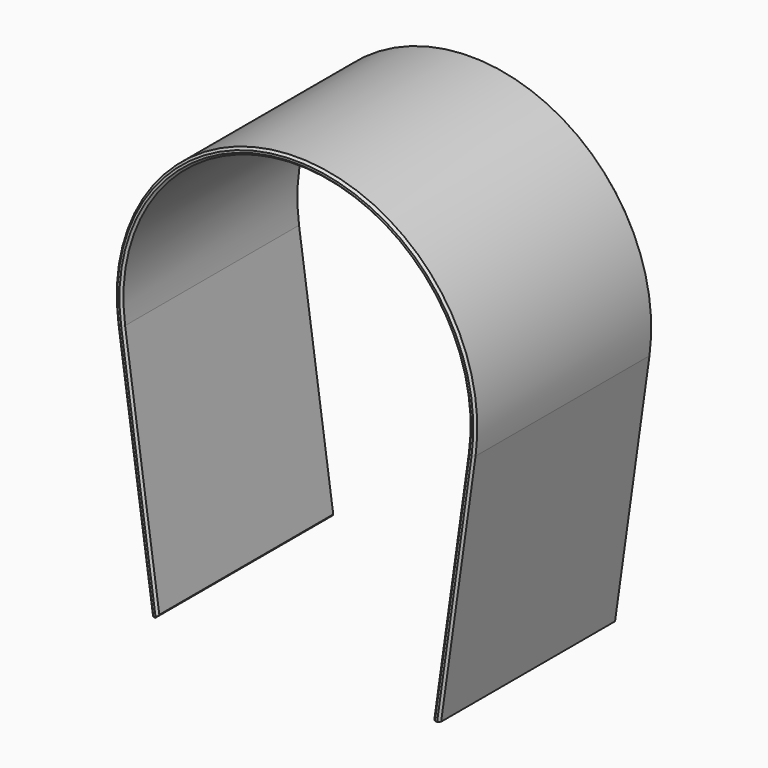
from build123d import *

# Parameters (mm, degrees)
F1_DEPTH     = 100
F2_T1_DEPTH  = 105.8849898869
F2_T3_DEPTH  = 114.5074829388
F2_T5_DEPTH  = 114.0858604347
F2_T7_DEPTH  = 114.5074829388
F2_T9_DEPTH  = 114.0858604347
F2_T12_ANGLE = 196
F2_T14_ANGLE = 196
F2_T16_ANGLE = 196
F2_T18_ANGLE = 196


# Not quite as in the source:
# - a fillet or chamfer that OpenCascade refuses, or shapes differently, is made with other operations: its cross-section is extruded or revolved along the edge and cut away or added


with BuildPart() as f1:
    # F0 (on Front) → F1 (new body)
    with BuildSketch(Plane.XZ):
        with BuildLine():
            Line((-61.9215476124, -110.8464484404), (-77.5, 0))
            ThreePointArc((-77.5, 0), (0, 89.1535515596), (77.5, 0))
            Line((77.5, 0), (61.9215476124, -110.8464484404))
            Line((61.9215476124, -110.8464484404), (64.95103033, -110.8464484404))
            Line((64.95103033, -110.8464484404), (80.4708042062, -0.4175193029))
            ThreePointArc((80.4708042062, -0.4175193029), (0, 92.1535515596), (-80.4708042062, -0.4175193029))
            Line((-80.4708042062, -0.4175193029), (-64.95103033, -110.8464484404))
            Line((-64.95103033, -110.8464484404), (-61.9215476124, -110.8464484404))
        make_face()
    extrude(amount=F1_DEPTH)

    # F2: chamfer of 1 on 17 edges, made by hand

    # F2_s2 → F2_t1 (cut)
    with BuildSketch(Plane.XZ.offset(-2.9424949434)):
        Polygon((-63.0719160196, -110.8464484404), (-62.0816479509, -109.7072753394), (-61.9215476124, -110.8464484404), align=None)
    extrude(amount=F2_T1_DEPTH, mode=Mode.SUBTRACT)

    # F2_s4 → F2_t3 (cut)
    with BuildSketch(Plane(origin=(14.4352522013, 0, -102.7121564484), x_dir=(0, 1, 0), z_dir=(-0.139173101, 0, 0.9902680687))):
        Polygon((-1, 76.7457753275), (0, 77.7457753275), (0, 76.7457753275), align=None)
        Polygon((-99, 76.7457753275), (-100, 77.7457753275), (-100, 76.7457753275), align=None)
    extrude(amount=F2_T3_DEPTH, mode=Mode.SUBTRACT)

    # F2_s6 → F2_t5 (cut)
    with BuildSketch(Plane(origin=(-1.5011092824, 0, 10.6809475379), x_dir=(0, 1, 0), z_dir=(0.139173101, 0, -0.9902680687))):
        Polygon((-1, -79.7457753275), (0, -78.7457753275), (0, -79.7457753275), align=None)
        Polygon((-99, -79.7457753275), (-100, -78.7457753275), (-100, -79.7457753275), align=None)
    extrude(amount=F2_T5_DEPTH, mode=Mode.SUBTRACT)

    # F2_s8 → F2_t7 (cut)
    with BuildSketch(Plane(origin=(1.5011092824, 0, 10.6809475379), x_dir=(0, 1, 0), z_dir=(-0.139173101, 0, -0.9902680687))):
        Polygon((-1, 76.7457753275), (0, 77.7457753275), (0, 76.7457753275), align=None)
        Polygon((-99, 76.7457753275), (-100, 77.7457753275), (-100, 76.7457753275), align=None)
    extrude(amount=F2_T7_DEPTH, mode=Mode.SUBTRACT)

    # F2_s10 → F2_t9 (cut)
    with BuildSketch(Plane(origin=(-14.37657369, 0, -102.2946371455), x_dir=(0, 1, 0), z_dir=(0.139173101, 0, 0.9902680687))):
        Polygon((-1, -79.7457753275), (0, -78.7457753275), (0, -79.7457753275), align=None)
        Polygon((-99, -79.7457753275), (-100, -78.7457753275), (-100, -79.7457753275), align=None)
    extrude(amount=F2_T9_DEPTH, mode=Mode.SUBTRACT)

    # F2_s11 → F2_t12 (revolve, cut)
    with BuildSketch(Plane(origin=(1.5011092824, 0, 10.6809475379), x_dir=(0, 1, 0), z_dir=(-0.139173101, 0, -0.9902680687))):
        Polygon((-1, 79.7457753275), (0, 78.7457753275), (0, 79.7457753275), align=None)
    revolve(axis=Axis((0, 0, 10.8919146894), (0, -1, 0)), revolution_arc=F2_T12_ANGLE, mode=Mode.SUBTRACT)

    # F2_s13 → F2_t14 (revolve, cut)
    with BuildSketch(Plane(origin=(1.5011092824, 0, 10.6809475379), x_dir=(0, 1, 0), z_dir=(-0.139173101, 0, -0.9902680687))):
        Polygon((-99, 79.7457753275), (-100, 78.7457753275), (-100, 79.7457753275), align=None)
    revolve(axis=Axis((0, -100, 10.8919146894), (0, -1, 0)), revolution_arc=F2_T14_ANGLE, mode=Mode.SUBTRACT)

    # F2_s15 → F2_t16 (revolve, cut)
    with BuildSketch(Plane(origin=(-1.5011092824, 0, 10.6809475379), x_dir=(0, 1, 0), z_dir=(0.139173101, 0, -0.9902680687))):
        Polygon((-1, -76.7457753275), (0, -77.7457753275), (0, -76.7457753275), align=None)
    revolve(axis=Axis((0, 0, 10.8919146894), (0, 1, 0)), revolution_arc=F2_T16_ANGLE, mode=Mode.SUBTRACT)

    # F2_s17 → F2_t18 (revolve, cut)
    with BuildSketch(Plane(origin=(-1.5011092824, 0, 10.6809475379), x_dir=(0, 1, 0), z_dir=(0.139173101, 0, -0.9902680687))):
        Polygon((-99, -76.7457753275), (-100, -77.7457753275), (-100, -76.7457753275), align=None)
    revolve(axis=Axis((0, -100, 10.8919146894), (0, 1, 0)), revolution_arc=F2_T18_ANGLE, mode=Mode.SUBTRACT)


solid = f1.part
